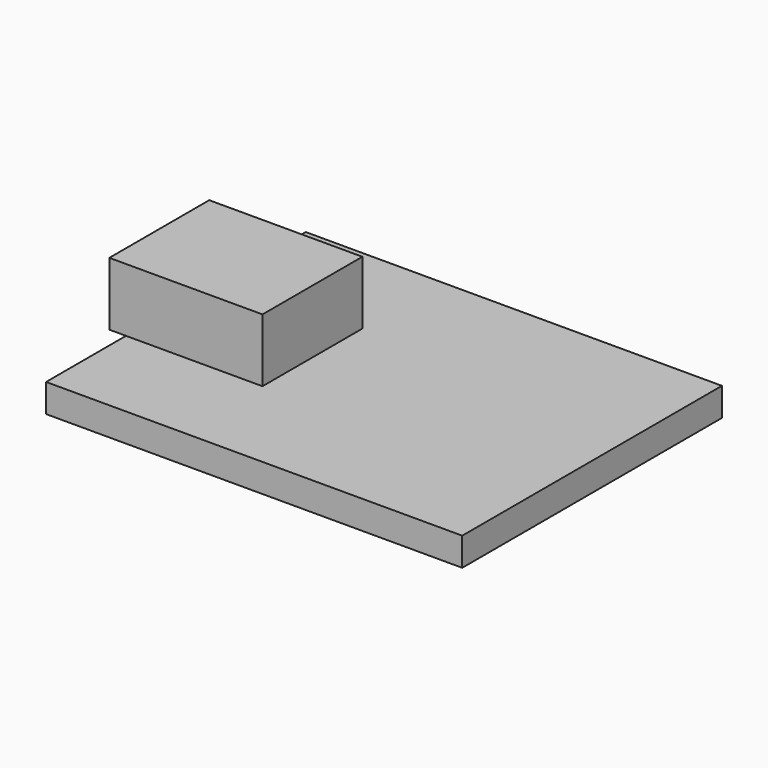
from build123d import *

# Parameters (mm, degrees)
F0_W     = 25
F0_H     = 19.5
F1_DEPTH = 1.7
F2_W     = 9.2
F2_H     = 7.5
F3_DEPTH = 3.8


# Not quite as in the source:
# - a feature names something its author has since deleted; it is built from what else it names


with BuildPart() as f1:
    # F0 (on Top) → F1 (new body)
    with BuildSketch(Plane.XY):
        Rectangle(F0_W, F0_H)
    extrude(amount=F1_DEPTH)

    # F2 (on face) → F3 (join)
    with BuildSketch(Plane.XY.offset(1.7)):
        with Locations((-8.9, 0)):
            Rectangle(F2_W, F2_H)
    extrude(amount=F3_DEPTH)


solid = f1.part
